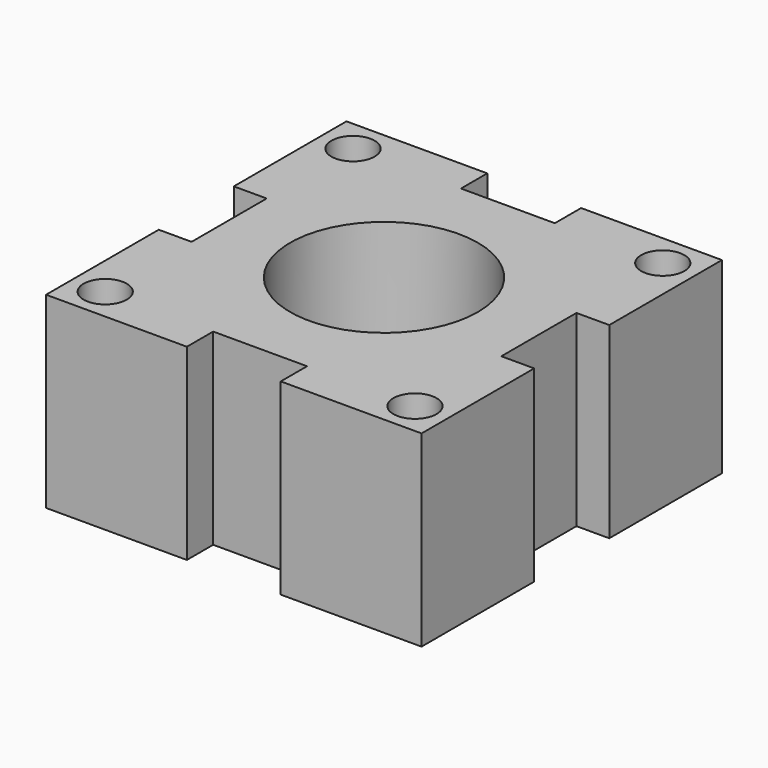
from build123d import *

# Parameters (mm, degrees)
F0_R     = 2.921
F0_R_2   = 12.7
F1_DEPTH = 25.4


# Not quite as in the source:
# - the program builds the solid bodies; features that only make, move or delete a surface that nothing else refers to are left out


with BuildPart() as f1:
    # F0 (on Top) → F1 (new body)
    with BuildSketch(Plane.XY):
        Polygon((31.1358614907, 25.4), (12.0858614907, 25.4), (12.0858614907, 6.35), (16.5308614907, 6.35), (16.5308614907, -6.35), (12.0858614907, -6.35), (12.0858614907, -25.4), (31.1358614907, -25.4), (31.1358614907, -20.955), (43.8358614907, -20.955), (43.8358614907, -25.4), (62.8858614907, -25.4), (62.8858614907, -6.35), (58.4408614907, -6.35), (58.4408614907, 6.35), (62.8858614907, 6.35), (62.8858614907, 25.4), (43.8358614907, 25.4), (43.8358614907, 20.955), (31.1358614907, 20.955), align=None)
        with Locations((16.5308614907, -20.955)):
            Circle(F0_R, mode=Mode.SUBTRACT)
        with Locations((37.4858614907, 0)):
            Circle(F0_R_2, mode=Mode.SUBTRACT)
        with Locations((58.4408614907, -20.955)):
            Circle(F0_R, mode=Mode.SUBTRACT)
        with Locations((16.5308614907, 20.955)):
            Circle(F0_R, mode=Mode.SUBTRACT)
        with Locations((58.4408614907, 20.955)):
            Circle(F0_R, mode=Mode.SUBTRACT)
    extrude(amount=F1_DEPTH)


solid = f1.part
